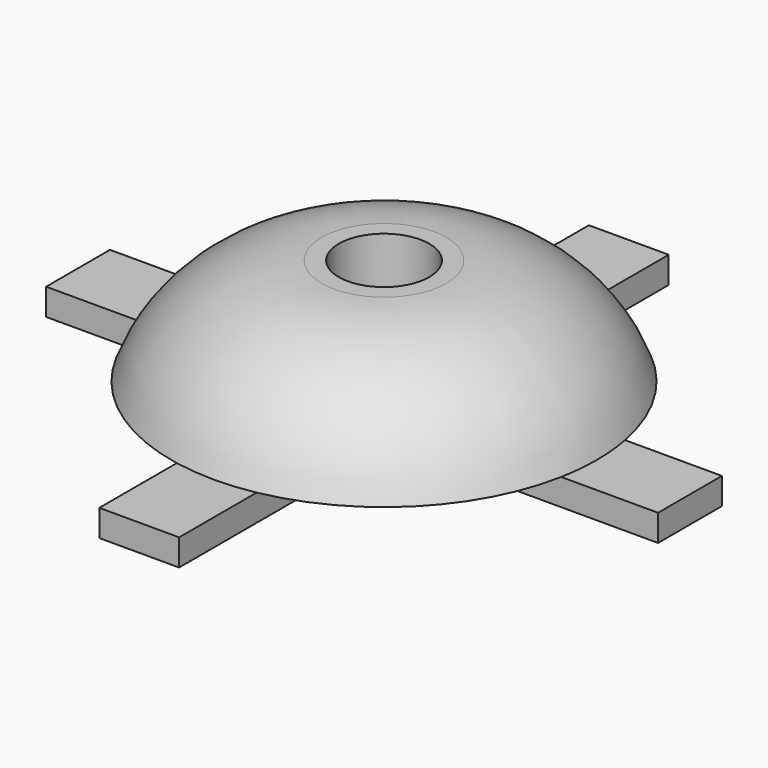
from build123d import *

# Parameters (mm, degrees)
F0_W     = 19.05
F0_H     = 63.5
F0_W_2   = 63.5
F0_H_2   = 19.05
F1_DEPTH = 6.35
F2_R     = 10.795
F3_DEPTH = 25.4
F4_DEPTH = 6.35


# Not quite as in the source:
# - a fillet or chamfer that OpenCascade refuses, or shapes differently, is made with other operations: its cross-section is extruded or revolved along the edge and cut away or added


with BuildPart() as f1:
    # F0 (on Top) → F1 (new body)
    with BuildSketch(Plane.XY):
        with Locations((0, 41.275)):
            Rectangle(F0_W, F0_H)
        with Locations((-41.275, 0)):
            Rectangle(F0_W_2, F0_H_2)
        Rectangle(F0_W, F0_H_2)
        with Locations((41.275, 0)):
            Rectangle(F0_W_2, F0_H_2)
        with Locations((0, -41.275)):
            Rectangle(F0_W, F0_H)
    extrude(amount=F1_DEPTH)

    # F2 (on face) → F3 (join)
    with BuildSketch(Plane.XY.offset(6.35)):
        with BuildLine():
            ThreePointArc((49.8990418245, -9.525), (50.5742588907, -4.7837576923), (50.8, 0))
            ThreePointArc((50.8, 0), (50.5742588907, 4.7837576923), (49.8990418245, 9.525))
            Line((49.8990418245, 9.525), (9.525, 9.525))
            Line((9.525, 9.525), (9.525, 49.8990418245))
            ThreePointArc((9.525, 49.8990418245), (0, 50.8), (-9.525, 49.8990418245))
            Line((-9.525, 49.8990418245), (-9.525, 9.525))
            Line((-9.525, 9.525), (-49.8990418245, 9.525))
            ThreePointArc((-49.8990418245, 9.525), (-50.8, 0), (-49.8990418245, -9.525))
            Line((-49.8990418245, -9.525), (-9.525, -9.525))
            Line((-9.525, -9.525), (-9.525, -49.8990418245))
            ThreePointArc((-9.525, -49.8990418245), (0, -50.8), (9.525, -49.8990418245))
            Line((9.525, -49.8990418245), (9.525, -9.525))
            Line((9.525, -9.525), (49.8990418245, -9.525))
        make_face()
        Circle(F2_R, mode=Mode.SUBTRACT)
        with BuildLine():
            ThreePointArc((-49.8990418245, -9.525), (-35.9210244843, -35.9210244843), (-9.525, -49.8990418245))
            Line((-9.525, -49.8990418245), (-9.525, -9.525))
            Line((-9.525, -9.525), (-49.8990418245, -9.525))
        make_face()
        with BuildLine():
            Line((-9.525, 9.525), (-9.525, 49.8990418245))
            ThreePointArc((-9.525, 49.8990418245), (-35.9210244843, 35.9210244843), (-49.8990418245, 9.525))
            Line((-49.8990418245, 9.525), (-9.525, 9.525))
        make_face()
        with BuildLine():
            Line((9.525, 9.525), (49.8990418245, 9.525))
            ThreePointArc((49.8990418245, 9.525), (35.9210244843, 35.9210244843), (9.525, 49.8990418245))
            Line((9.525, 49.8990418245), (9.525, 9.525))
        make_face()
        with BuildLine():
            ThreePointArc((9.525, -49.8990418245), (35.9210244843, -35.9210244843), (49.8990418245, -9.525))
            Line((49.8990418245, -9.525), (9.525, -9.525))
            Line((9.525, -9.525), (9.525, -49.8990418245))
        make_face()
    extrude(amount=F3_DEPTH)

    # F4 (cut, through all): a face of the model
    f4_faces = [f1.faces().sort_by_distance(p)[0] for p in [
        (0, 0, 6.35),
    ]]
    extrude(f4_faces, amount=-F4_DEPTH, mode=Mode.SUBTRACT)

    # F5: fillet of radius 38.1 on 1 edges, made by hand

    # F5_s1 → F5_t2 (revolve, cut)
    with BuildSketch(Plane(origin=(0, 0, 0), x_dir=(0, 0, 1), z_dir=(-0.9822646028, -0.1875, 0))):
        with BuildLine():
            ThreePointArc((6.35, -50.8), (24.7585197333, -36.8760207718), (31.75, -14.8789755157))
            Line((31.75, -14.8789755157), (32.512, -14.8789755157))
            Line((32.512, -14.8789755157), (32.512, -50.8))
            Line((32.512, -50.8), (31.75, -51.562))
            ThreePointArc((31.75, -51.562), (19.05, -51.562), (6.604, -51.5184204897))
            Line((6.604, -51.5184204897), (6.35, -50.8))
        make_face()
    revolve(axis=Axis((0, 0, 31.75), (0, 0, 1)), mode=Mode.SUBTRACT)


solid = f1.part
